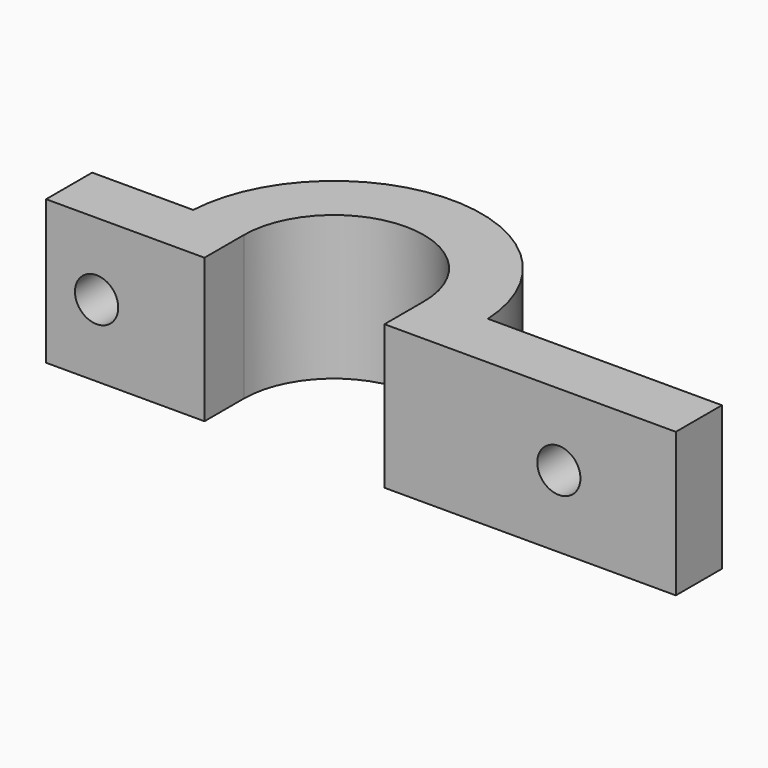
from build123d import *

# Parameters (mm, degrees)
F1_DEPTH  = 10
F3_DEPTH  = 13.6785106988
F4_DEPTH  = 3.268
F6_DEPTH  = 4
F8_DEPTH  = 4
F9_R      = 1.5
F10_DEPTH = 4.001


# Not quite as in the source:
# - a feature names something its author has since deleted; it is built from what else it names


with BuildPart() as f1:
    # F0 (on Top) → F1 (new body)
    with BuildSketch(Plane.XY):
        with BuildLine():
            Line((14.6115271971, -9.8928403326), (14.6115271971, -13.3118403326))
            Line((14.6115271971, -13.3118403326), (38.1115271971, -13.3118403326))
            Line((38.1115271971, -13.3118403326), (38.1115271971, -9.3118403326))
            Line((38.1115271971, -9.3118403326), (18.5955271971, -9.3118403326))
            ThreePointArc((18.5955271971, -9.3118403326), (8.3615271971, 0.3656703662), (-1.8724728029, -9.3118403326))
            Line((-1.8724728029, -9.3118403326), (-8.8884728029, -9.3118403326))
            Line((-8.8884728029, -9.3118403326), (-8.8884728029, -13.3118403326))
            Line((-8.8884728029, -13.3118403326), (2.1115271971, -13.3118403326))
            Line((2.1115271971, -13.3118403326), (2.1115271971, -9.8928403326))
            ThreePointArc((2.1115271971, -9.8928403326), (8.3615271971, -3.6428403326), (14.6115271971, -9.8928403326))
        make_face()
    extrude(amount=F1_DEPTH)

    # F2 (on face) → F3 (cut, through all)
    with BuildSketch(Plane.XZ.offset(13.3118403326)):
        Polygon((-2.1564728029, 5), (-3.0224728029, 6.4999559994), (-4.7544728029, 6.4999559994), (-5.6204728029, 5), (-4.7544728029, 3.5000440006), (-3.0224728029, 3.5000440006), align=None)
        Polygon((29.9775271971, 6.4999559994), (28.2455271971, 6.4999559994), (27.3795271971, 5), (28.2455271971, 3.5000440006), (29.9775271971, 3.5000440006), (30.8435271971, 5), align=None)
    extrude(amount=-F3_DEPTH, mode=Mode.SUBTRACT)

    # F4 (cut): a face of the model
    f4_faces = [f1.faces().sort_by_distance(p)[0] for p in [
        (38.1115271971, -11.3118403326, 5),
    ]]
    extrude(f4_faces, amount=-F4_DEPTH, mode=Mode.SUBTRACT)

    # F5 (on face) → F6 (join, through all)
    with BuildSketch(Plane(origin=(0, -9.3118403326, 0), x_dir=(-1, 0, 0), z_dir=(0, 1, 0))):
        Polygon((4.7544728029, 3.5000440006), (5.6204728029, 5), (4.7544728029, 6.4999559994), (3.0224728029, 6.4999559994), (2.1564728029, 5), (3.0224728029, 3.5000440006), align=None)
    extrude(amount=-F6_DEPTH)

    # F7 (on face) → F8 (join, through all)
    with BuildSketch(Plane(origin=(0, -9.3118403326, 0), x_dir=(-1, 0, 0), z_dir=(0, 1, 0))):
        Polygon((-28.2455271971, 3.5000440006), (-27.3795271971, 5), (-28.2455271971, 6.4999559994), (-29.9775271971, 6.4999559994), (-30.8435271971, 5), (-29.9775271971, 3.5000440006), align=None)
    extrude(amount=-F8_DEPTH)

    # F9 (on face) → F10 (cut, through all)
    with BuildSketch(Plane(origin=(0, -9.3118403326, 0), x_dir=(-1, 0, 0), z_dir=(0, 1, 0))):
        with Locations((5.3804728029, 5)):
            Circle(F9_R)
        with Locations((-26.7195271971, 5)):
            Circle(F9_R)
    extrude(amount=-F10_DEPTH, mode=Mode.SUBTRACT)


solid = f1.part
